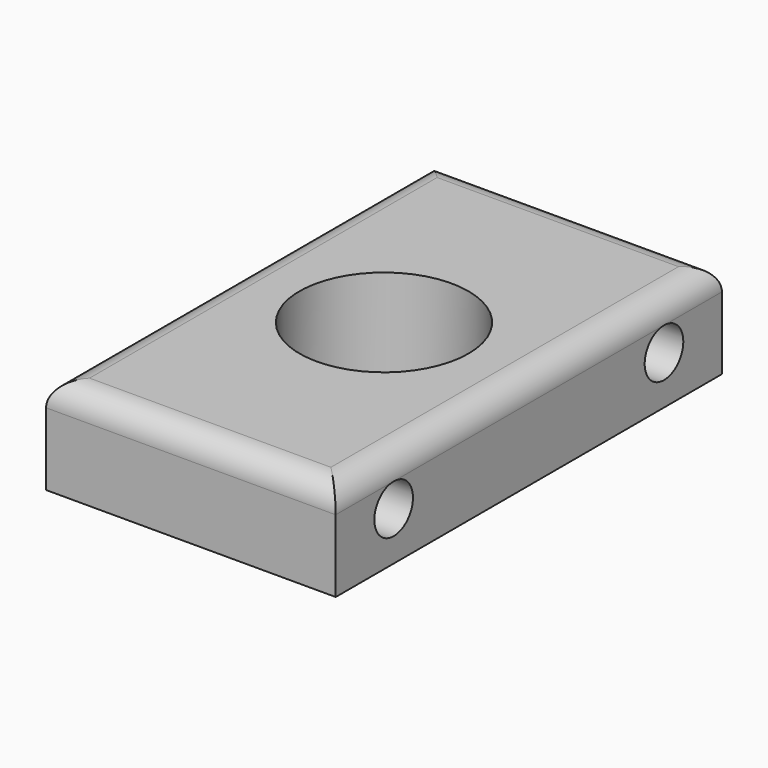
from build123d import *

# Parameters (mm, degrees)
F0_W     = 60
F0_H     = 100
F0_R     = 17.5
F1_DEPTH = 20
F2_W     = 100
F2_H     = 20
F2_R     = 5
F3_DEPTH = 100
F4_R     = 4.99999


# Not quite as in the source:
# - a fillet or chamfer is up to 0.001 mm smaller than in the source, because OpenCascade refuses the exact size


with BuildPart() as f1:
    # F0 (on Top) → F1 (new body)
    with BuildSketch(Plane.XY):
        Rectangle(F0_W, F0_H)
        Circle(F0_R, mode=Mode.SUBTRACT)
    extrude(amount=F1_DEPTH)

    # F2 (on face) → F3 (intersect)
    with BuildSketch(Plane.YZ.offset(30)):
        with Locations((0, 10)):
            Rectangle(F2_W, F2_H)
        with Locations((-35, 10)):
            Circle(F2_R, mode=Mode.SUBTRACT)
        with Locations((35, 10)):
            Circle(F2_R, mode=Mode.SUBTRACT)
    extrude(amount=-F3_DEPTH, mode=Mode.INTERSECT)

    # F4 (radius 5 in the source; OpenCascade refuses exactly that, so slightly less here)
    f4_edges = [f1.edges().sort_by_distance(p)[0] for p in [
        (30, 0, 20),
        (0, -50, 20),
        (-30, 0, 20),
        (0, 50, 20),
    ]]
    fillet(f4_edges, radius=F4_R)


solid = f1.part
